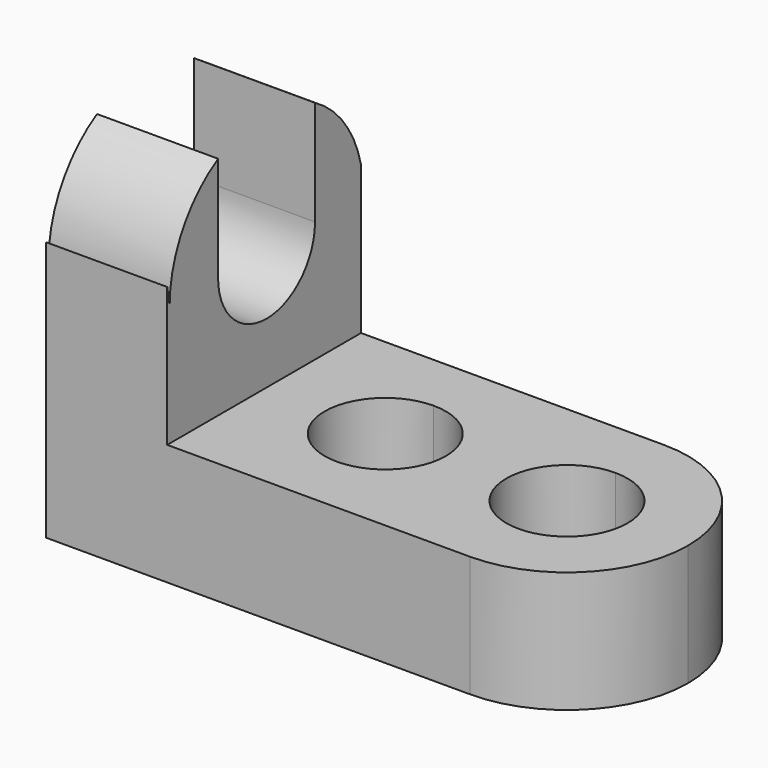
from build123d import *

# Parameters (mm, degrees)
F1_DEPTH = 25.4
F3_DEPTH = 25.4
F5_DEPTH = 25.4


# Not quite as in the source:
# - a feature names something its author has since deleted; it is built from what else it names


with BuildPart() as f1:
    # F0 (on Front) → F1 (new body)
    with BuildSketch(Plane.XZ):
        Polygon((0, 38.1), (0, 0), (57.15, 0), (57.15, 12.7), (12.7, 12.7), (12.7, 38.1), align=None)
    extrude(amount=F1_DEPTH)

    # F2 (on Top) → F3 (cut)
    with BuildSketch(Plane.XY):
        with BuildLine():
            Line((25.4, -19.05), (25.4, -6.35))
            ThreePointArc((25.4, -6.35), (19.05, -12.7), (25.4, -19.05))
        make_face()
        with BuildLine():
            ThreePointArc((25.4, -19.05), (29.8901280605, -17.1901280605), (31.75, -12.7))
            ThreePointArc((31.75, -12.7), (29.8901280605, -8.2098719395), (25.4, -6.35))
            Line((25.4, -6.35), (25.4, -19.05))
        make_face()
        with BuildLine():
            Line((44.45, -19.05), (44.45, -6.35))
            ThreePointArc((44.45, -6.35), (38.1, -12.7), (44.45, -19.05))
        make_face()
        with BuildLine():
            ThreePointArc((50.8, -12.7), (48.9401280605, -8.2098719395), (44.45, -6.35))
            Line((44.45, -6.35), (44.45, -19.05))
            ThreePointArc((44.45, -19.05), (48.9401280605, -17.1901280605), (50.8, -12.7))
        make_face()
        with BuildLine():
            Line((57.15, -25.4), (57.15, -12.7))
            ThreePointArc((57.15, -12.7), (53.4302561211, -21.6802561211), (44.45, -25.4))
            Line((44.45, -25.4), (57.15, -25.4))
        make_face()
        with BuildLine():
            Line((57.15, 0), (44.45, 0))
            ThreePointArc((44.45, 0), (53.4302561211, -3.7197438789), (57.15, -12.7))
            Line((57.15, -12.7), (57.15, 0))
        make_face()
    extrude(amount=F3_DEPTH, mode=Mode.SUBTRACT)

    # F4 (on Right) → F5 (cut)
    with BuildSketch(Plane.YZ):
        with BuildLine():
            ThreePointArc((-18.7333624887, 25.4), (-12.3833624887, 19.05), (-6.0333624887, 25.4))
            ThreePointArc((-6.0333624887, 25.4), (-12.3833624887, 31.75), (-18.7333624887, 25.4))
        make_face()
        with BuildLine():
            ThreePointArc((-18.7333624887, 25.4), (-12.3833624887, 31.75), (-6.0333624887, 25.4))
            Line((-6.0333624887, 25.4), (-6.0333624887, 36.3985226281))
            ThreePointArc((-6.0333624887, 36.3985226281), (-9.0963606159, 37.6672579939), (-12.3833624887, 38.1))
            ThreePointArc((-12.3833624887, 38.1), (-15.6703643615, 37.6672579939), (-18.7333624887, 36.3985226281))
            Line((-18.7333624887, 36.3985226281), (-18.7333624887, 25.4))
        make_face()
        with BuildLine():
            ThreePointArc((-12.3833624887, 38.1), (-9.0963606159, 37.6672579939), (-6.0333624887, 36.3985226281))
            Line((-6.0333624887, 36.3985226281), (-6.0333624887, 38.1))
            Line((-6.0333624887, 38.1), (-12.3833624887, 38.1))
        make_face()
        with BuildLine():
            Line((-6.0333624887, 38.1), (-6.0333624887, 36.3985226281))
            ThreePointArc((-6.0333624887, 36.3985226281), (-1.3848398607, 31.75), (0.3166375113, 25.4))
            Line((0.3166375113, 25.4), (0.3166375113, 40.4268426491))
            Line((0.3166375113, 40.4268426491), (-27.6233624887, 40.4268426491))
            Line((-27.6233624887, 40.4268426491), (-25.0833624887, 25.4))
            ThreePointArc((-25.0833624887, 25.4), (-23.3818851168, 31.75), (-18.7333624887, 36.3985226281))
            Line((-18.7333624887, 36.3985226281), (-18.7333624887, 38.1))
            Line((-18.7333624887, 38.1), (-12.3833624887, 38.1))
            Line((-12.3833624887, 38.1), (-6.0333624887, 38.1))
        make_face()
        with BuildLine():
            Line((-18.7333624887, 38.1), (-18.7333624887, 36.3985226281))
            ThreePointArc((-18.7333624887, 36.3985226281), (-15.6703643615, 37.6672579939), (-12.3833624887, 38.1))
            Line((-12.3833624887, 38.1), (-18.7333624887, 38.1))
        make_face()
    extrude(amount=F5_DEPTH, mode=Mode.SUBTRACT)


solid = f1.part
